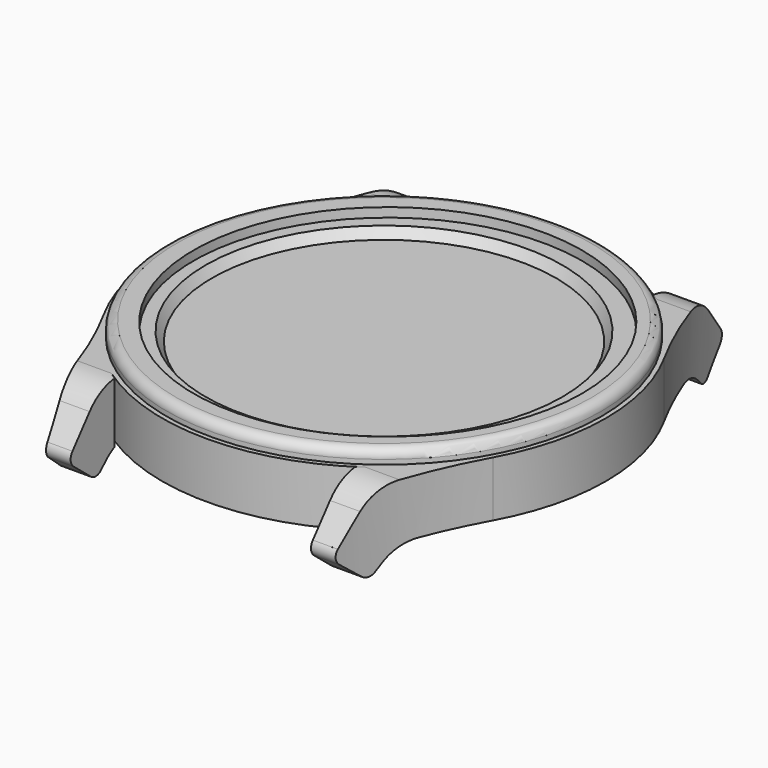
from build123d import *

# Parameters (mm, degrees)
F3_DEPTH      = 25
F6_DEPTH      = 25
F6_DEPTH_BACK = 25
F8_DEPTH      = 25
F8_DEPTH_BACK = 25
F10_R         = 24
F11_DEPTH     = 6
F13_DEPTH     = 1
F15_R         = 23.5
F16_DEPTH     = 1.5
F17_R         = 1
F18_R         = 20
F19_DEPTH     = 2
F19_TAPER     = 35
F20_R         = 21
F21_DEPTH     = 1


# Not quite as in the source:
# - a fillet or chamfer that OpenCascade refuses, or shapes differently, is made with other operations: its cross-section is extruded or revolved along the edge and cut away or added


with BuildPart() as f3:
    # F2 (on Top) → F3 (new body)
    with BuildSketch(Plane.XY):
        with BuildLine():
            Line((-13, 20.1742410018), (-13, 26.1742410018))
            Line((-13, 26.1742410018), (-15.6435015354, 26.1742410018))
            ThreePointArc((-15.6435015354, 26.1742410018), (-17.78469231, 18.672379989), (-21.0241029415, 11.5752795))
            ThreePointArc((-21.0241029415, 11.5752795), (-17.5469493067, 16.3738990478), (-13, 20.1742410018))
        make_face()
    extrude(amount=F3_DEPTH)


with BuildPart() as f3b:
    # F2 (on Top) → F3, piece 2 (new body)
    with BuildSketch(Plane.XY):
        with BuildLine():
            Line((13, 26.1742410018), (13, 20.1742410018))
            ThreePointArc((13, 20.1742410018), (17.5469493067, 16.3738990478), (21.0241029415, 11.5752795))
            ThreePointArc((21.0241029415, 11.5752795), (17.78469231, 18.672379989), (15.6435015354, 26.1742410018))
            Line((15.6435015354, 26.1742410018), (13, 26.1742410018))
        make_face()
    extrude(amount=F3_DEPTH)


with BuildPart() as f3c:
    # F2 (on Top) → F3, piece 3 (new body)
    with BuildSketch(Plane.XY):
        with BuildLine():
            ThreePointArc((-13, -20.1742410018), (-17.5469493067, -16.3738990478), (-21.0241029415, -11.5752795))
            ThreePointArc((-21.0241029415, -11.5752795), (-17.78469231, -18.672379989), (-15.6435015354, -26.1742410018))
            Line((-15.6435015354, -26.1742410018), (-13, -26.1742410018))
            Line((-13, -26.1742410018), (-13, -20.1742410018))
        make_face()
    extrude(amount=F3_DEPTH)


with BuildPart() as f3d:
    # F2 (on Top) → F3, piece 4 (new body)
    with BuildSketch(Plane.XY):
        with BuildLine():
            ThreePointArc((15.6435015354, -26.1742410018), (17.78469231, -18.672379989), (21.0241029415, -11.5752795))
            ThreePointArc((21.0241029415, -11.5752795), (17.5469493067, -16.3738990478), (13, -20.1742410018))
            Line((13, -20.1742410018), (13, -26.1742410018))
            Line((13, -26.1742410018), (15.6435015354, -26.1742410018))
        make_face()
    extrude(amount=F3_DEPTH)


with BuildPart() as f6_tool:
    # F5 (on Right) → F6 (new body, two sides)
    with BuildSketch(Plane.YZ) as f6_sk:
        with BuildLine():
            Line((23.5471649475, 7.1683851421), (27.7989016838, 1.9778330012))
            Line((27.7989016838, 1.9778330012), (27.7989016838, 26.740285454))
            Line((27.7989016838, 26.740285454), (-29.0615007661, 26.740285454))
            Line((-29.0615007661, 26.740285454), (-27.7989016838, 1.9778330012))
            Line((-27.7989016838, 1.9778330012), (-23.5471649475, 7.1683851421))
            ThreePointArc((-23.5471649475, 7.1683851421), (-21.8190448857, 8.5189558788), (-19.6791764535, 8.999999905))
            Line((-19.6791764535, 8.999999905), (0, 8.999999905))
            Line((0, 8.999999905), (19.6791764535, 8.999999905))
            ThreePointArc((19.6791764535, 8.999999905), (21.8190448857, 8.5189558788), (23.5471649475, 7.1683851421))
        make_face()
    extrude(amount=-F6_DEPTH)
    extrude(f6_sk.sketch, amount=F6_DEPTH_BACK)


with BuildPart() as f3_1:
    add(f3.part)

    # F6: cut by f6_tool
    add(f6_tool.part, mode=Mode.SUBTRACT)


with BuildPart() as f3b_1:
    add(f3b.part)

    # F6: cut by f6_tool
    add(f6_tool.part, mode=Mode.SUBTRACT)


with BuildPart() as f3c_1:
    add(f3c.part)

    # F6: cut by f6_tool
    add(f6_tool.part, mode=Mode.SUBTRACT)


with BuildPart() as f3d_1:
    add(f3d.part)

    # F6: cut by f6_tool
    add(f6_tool.part, mode=Mode.SUBTRACT)


with BuildPart() as f8_tool:
    # F7 (on Right) → F8 (new body, two sides)
    with BuildSketch(Plane.YZ) as f8_sk:
        with BuildLine():
            Line((17.8908835105, 3), (0, 3))
            Line((0, 3), (-17.8908835105, 3))
            ThreePointArc((-17.8908835105, 3), (-19.7544863974, 2.639718125), (-21.3495203475, 1.6107937119))
            Line((-21.3495203475, 1.6107937119), (-22.0408191574, 0.9486258563))
            ThreePointArc((-22.0408191574, 0.9486258563), (-22.6937657116, 0.6715368573), (-23.3662235722, 0.8971868999))
            Line((-23.3662235722, 0.8971868999), (-25.727452218, 2.8313400119))
            ThreePointArc((-25.727452218, 2.8313400119), (-26.1117766069, 3.5541907786), (-25.8675033398, 4.3355671527))
            Line((-25.8675033398, 4.3355671527), (-26.6892556101, 5.8121909387))
            Line((-26.6892556101, 5.8121909387), (-28.4930374473, 3.2282707538))
            Line((-28.4930374473, 3.2282707538), (-28.1138848513, -2.6890258305))
            Line((-28.1138848513, -2.6890258305), (27.818409726, -2.2570919245))
            Line((27.818409726, -2.2570919245), (26.8063536115, 3.2282707538))
            Line((26.8063536115, 3.2282707538), (26.1989608407, 4.4945557602))
            Line((26.1989608407, 4.4945557602), (25.8675033398, 4.3355671527))
            ThreePointArc((25.8675033398, 4.3355671527), (26.1117766069, 3.5541907786), (25.727452218, 2.8313400119))
            Line((25.727452218, 2.8313400119), (23.3662235722, 0.8971868999))
            ThreePointArc((23.3662235722, 0.8971868999), (22.6937657116, 0.6715368573), (22.0408191574, 0.9486258563))
            Line((22.0408191574, 0.9486258563), (21.3495203475, 1.6107937119))
            ThreePointArc((21.3495203475, 1.6107937119), (19.7544863974, 2.639718125), (17.8908835105, 3))
        make_face()
    extrude(amount=-F8_DEPTH)
    extrude(f8_sk.sketch, amount=F8_DEPTH_BACK)


with BuildPart() as f3_2:
    add(f3_1.part)

    # F8: cut by f8_tool
    add(f8_tool.part, mode=Mode.SUBTRACT)



with BuildPart() as f3b_2:
    add(f3b_1.part)

    # F8: cut by f8_tool
    add(f8_tool.part, mode=Mode.SUBTRACT)


with BuildPart() as f3c_2:
    add(f3c_1.part)

    # F8: cut by f8_tool
    add(f8_tool.part, mode=Mode.SUBTRACT)


with BuildPart() as f3d_2:
    add(f3d_1.part)

    # F8: cut by f8_tool
    add(f8_tool.part, mode=Mode.SUBTRACT)


with BuildPart() as f3_3:
    add(f3_2.part)

    add(f3b_2.part)  # F11 merges F3b

    add(f3c_2.part)  # F11 merges F3c

    add(f3d_2.part)  # F11 merges F3d
    # F10 (on plane+point) → F11 (join)
    with BuildSketch(Plane.XY.offset(3)):
        Circle(F10_R)
    extrude(amount=F11_DEPTH)

    # F12 (on face) → F13 (join)
    with BuildSketch(Plane(origin=(0, 0, 3), x_dir=(1, 0, 0), z_dir=(0, 0, -1))):
        with BuildLine():
            ThreePointArc((23, 0), (16.2634559673, 16.2634559673), (0, 23))
            ThreePointArc((0, 23), (-16.2634559673, 16.2634559673), (-23, 0))
            ThreePointArc((-23, 0), (-16.2634559673, -16.2634559673), (0, -23))
            ThreePointArc((0, -23), (16.2634559673, -16.2634559673), (23, 0))
        make_face()
    extrude(amount=F13_DEPTH)

    # F14: fillet of radius 5 on 1 edges, made by hand

    # F14_s1 → F14_t2 (revolve, cut)
    with BuildSketch(Plane.YZ):
        with BuildLine():
            ThreePointArc((23, 3), (21.5811388301, 2.2565835097), (20, 2))
            Line((20, 2), (23, 2))
            Line((23, 2), (23, 3))
        make_face()
    revolve(axis=Axis((0, 0, 2), (0, 0, 1)), mode=Mode.SUBTRACT)

    # F15 (on face) → F16 (join)
    with BuildSketch(Plane.XY.offset(8.999999905)):
        Circle(F15_R)
    extrude(amount=F16_DEPTH)

    # F17
    f17_edges = [f3_3.edges().sort_by_distance(p)[0] for p in [
        (-23.5, 0, 10.5),
    ]]
    fillet(f17_edges, radius=F17_R)

    # F18 (on face) → F19 (cut)
    with BuildSketch(Plane.XY.offset(10.499999905)):
        Circle(F18_R)
    extrude(amount=-F19_DEPTH, taper=F19_TAPER, mode=Mode.SUBTRACT)

    # F20 (on face) → F21 (cut)
    with BuildSketch(Plane.XY.offset(10.499999905)):
        with Locations((0.4080029248, 0)):
            Circle(F20_R)
    extrude(amount=-F21_DEPTH, mode=Mode.SUBTRACT)


solid = f3_3.part
